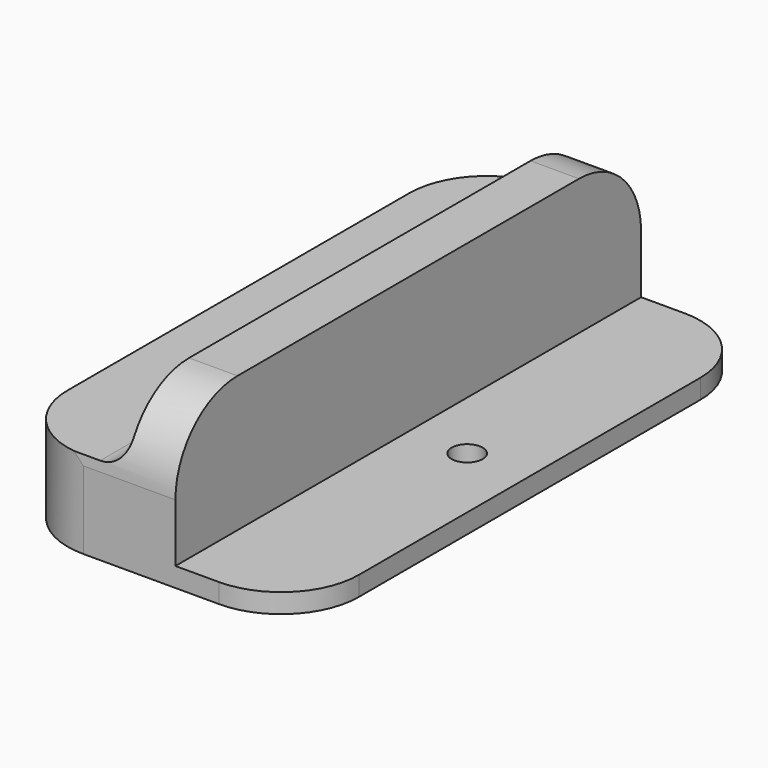
from build123d import *

# Parameters (mm, degrees)
F1_DEPTH    = 38.1
F2_R        = 1.778
F3_R        = 5.08
F4_R        = 1.016
F5_DEPTH    = 25.4
F6_T1_DEPTH = 28.575


# Not quite as in the source:
# - a fillet or chamfer that OpenCascade refuses, or shapes differently, is made with other operations: its cross-section is extruded or revolved along the edge and cut away or added


with BuildPart() as f1:
    # F0 (on Front) → F1 (new body)
    with BuildSketch(Plane.XZ):
        Polygon((0, 5.715), (0, 0), (19.05, 0), (19.05, 1.27), (11.1125, 1.27), (11.1125, 10.16), (7.9375, 10.16), (7.9375, 5.715), align=None)
    extrude(amount=F1_DEPTH)

    # F2
    f2_edges = [f1.edges().sort_by_distance(p)[0] for p in [
        (7.9375, -19.05, 5.715),
    ]]
    fillet(f2_edges, radius=F2_R)

    # F3
    f3_edges = [f1.edges().sort_by_distance(p)[0] for p in [
        (19.05, -38.1, 0.635),
        (0, -38.1, 2.8575),
        (0, 0, 2.8575),
        (19.05, 0, 0.635),
    ]]
    fillet(f3_edges, radius=F3_R)

    # F4 (on face) → F5 (cut)
    with BuildSketch(Plane.XY.offset(1.27)):
        with Locations((14.9681093171, -19.05)):
            Circle(F4_R)
    extrude(amount=-F5_DEPTH, mode=Mode.SUBTRACT)

    # F6: fillet of radius 5.08 on 2 edges, made by hand

    # F6_s2 → F6_t1 (cut)
    with BuildSketch(Plane.YZ.offset(-4.7625)):
        with BuildLine():
            ThreePointArc((-33.02, 10.16), (-36.6121024484, 8.6721024484), (-38.1, 5.08))
            Line((-38.1, 5.08), (-38.1, 10.16))
            Line((-38.1, 10.16), (-33.02, 10.16))
        make_face()
        with BuildLine():
            ThreePointArc((0, 5.08), (-1.4878975516, 8.6721024484), (-5.08, 10.16))
            Line((-5.08, 10.16), (0, 10.16))
            Line((0, 10.16), (0, 5.08))
        make_face()
    extrude(amount=F6_T1_DEPTH, mode=Mode.SUBTRACT)


solid = f1.part
